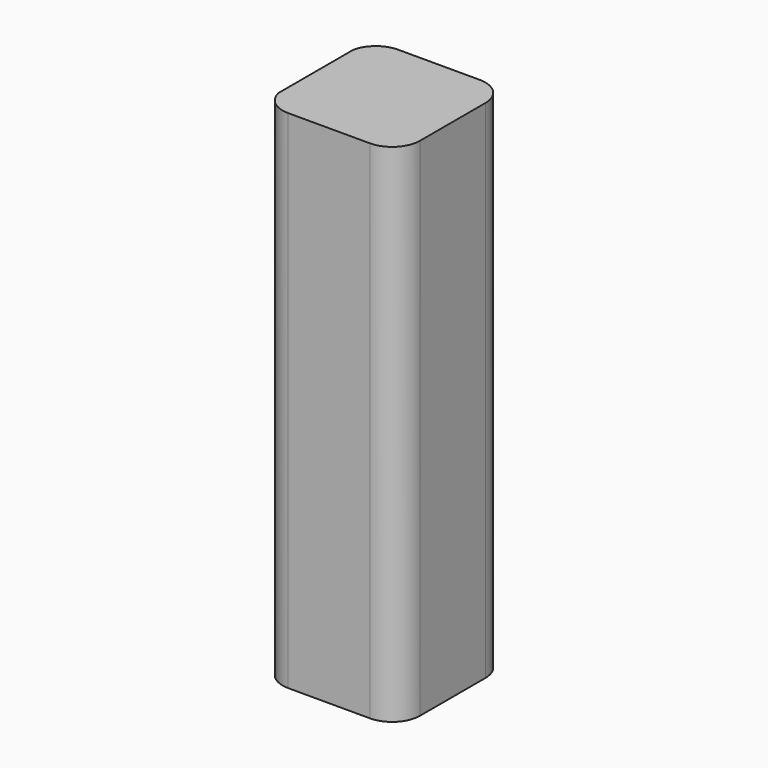
from build123d import *

# Parameters (mm, degrees)
F0_W         = 80
F0_H         = 60
F1_DEPTH     = 130
F2_T         = -1.5
F3_W         = 1.5
F3_H         = 27
F4_DEPTH     = 91
F5_R         = 1
F6_W         = 17
F6_H         = 16
F6_W_2       = 1.5
F6_H_2       = 27
F7_DEPTH     = 2
F8_T1_DEPTH  = 92
F8_T3_DEPTH  = 29.9726896882
F8_S7_W      = 1
F8_S7_H      = 1
F8_T8_DEPTH  = 1
F8_T15_DEPTH = 29.9726896882
F8_T19_DEPTH = 94.5
F9_T1_DEPTH  = 127.5
F9_T3_DEPTH  = 58.5
F9_S7_W      = 1
F9_S7_H      = 1
F9_T8_DEPTH  = 1
F9_S13_W     = 1
F9_S13_H     = 1
F9_T14_DEPTH = 1
F9_T18_ANGLE = 90
F11_DEPTH    = 60
F12_DEPTH    = 60
F13_DEPTH    = 50
F14_R        = 2
F15_W        = 17
F15_H        = 16
F16_DEPTH    = 91


# Not quite as in the source:
# - a fillet or chamfer that OpenCascade refuses, or shapes differently, is made with other operations: its cross-section is extruded or revolved along the edge and cut away or added


with BuildPart() as f1:
    # F0 (on Top) → F1 (new body)
    with BuildSketch(Plane.XY):
        Rectangle(F0_W, F0_H)
    extrude(amount=F1_DEPTH)

    # F2
    f2_openings = [f1.faces().sort_by_distance(p)[0] for p in [
        (0, 0, 130),
    ]]
    offset(amount=F2_T, openings=f2_openings)

    # F3 (on face) → F4 (join)
    with BuildSketch(Plane.XY.offset(1.5)):
        with Locations((11.75, -15)):
            Rectangle(F3_W, F3_H)
    extrude(amount=F4_DEPTH)

    # F5
    f5_edges = [f1.edges().sort_by_distance(p)[0] for p in [
        (0, 28.5, 1.5),
        (-38.5, 0, 1.5),
        (-13.75, -28.5, 1.5),
        (11, -15, 1.5),
    ]]
    fillet(f5_edges, radius=F5_R)

    # F6 (on face) → F7 (join)
    with BuildSketch(Plane.XY.offset(92.5)):
        Polygon((38.4726896882, -1.5), (12.5, -1.5), (12.5, -28.5), (11, -28.5), (11, -28.532365337), (38.4726896882, -28.532365337), align=None)
        with Locations((24.7363448441, -15)):
            Rectangle(F6_W, F6_H, mode=Mode.SUBTRACT)
        with Locations((11.75, -15)):
            Rectangle(F6_W_2, F6_H_2)
    extrude(amount=F7_DEPTH)

    # F8: fillet of radius 1 on 2 edges, made by hand

    # F8_s2 → F8_t1 (join)
    with BuildSketch(Plane.XY.offset(2.5)):
        with BuildLine():
            ThreePointArc((10, -28.5), (10.7071067812, -28.2071067812), (11, -27.5))
            Line((11, -27.5), (11, -28.5))
            Line((11, -28.5), (10, -28.5))
        make_face()
    extrude(amount=F8_T1_DEPTH)

    # F8_s4 → F8_t3 (join)
    with BuildSketch(Plane.YZ.offset(11)):
        with BuildLine():
            ThreePointArc((-28.5, 95.5), (-28.2071067812, 94.7928932188), (-27.5, 94.5))
            Line((-27.5, 94.5), (-28.5, 94.5))
            Line((-28.5, 94.5), (-28.5, 95.5))
        make_face()
    extrude(amount=F8_T3_DEPTH)


with BuildPart() as f8_tool6:
    # F8_s7 → F8_t8 (new body)
    with BuildSketch(Plane.XZ.offset(27.5)):
        with Locations((10.5, 2)):
            Rectangle(F8_S7_W, F8_S7_H)
    extrude(amount=F8_T8_DEPTH)

    # F8_s9 → F8_t10 (revolve, cut)
    with BuildSketch(Plane(origin=(10, -27.5, 2.5), x_dir=(-0.7071067812, 0, 0.7071067812), z_dir=(0.7071067812, 0, 0.7071067812))):
        with BuildLine():
            ThreePointArc((0, -1), (1, 0), (0, 1))
            Line((0, 1), (0, -1))
        make_face()
    revolve(axis=Axis((10, -27.5, 2.5), (0, -1, 0)), mode=Mode.SUBTRACT)


with BuildPart() as f1_1:
    add(f1.part)

    # F8_t5: union F8_tool6
    add(f8_tool6.part)


with BuildPart() as f8_tool13:
    # F8_s14 → F8_t15 (new body)
    with BuildSketch(Plane.YZ.offset(8.5)):
        with BuildLine():
            ThreePointArc((-28.5, 95.5), (-28.2071067812, 94.7928932188), (-27.5, 94.5))
            Line((-27.5, 94.5), (-28.5, 94.5))
            Line((-28.5, 94.5), (-28.5, 95.5))
        make_face()
    extrude(amount=F8_T15_DEPTH)

    split(bisect_by=Plane.YZ.offset(11), keep=Keep.BOTTOM)


with BuildPart() as f8_tool17:
    # F8_s18 → F8_t19 (new body)
    with BuildSketch(Plane.XY.offset(97)):
        with BuildLine():
            ThreePointArc((10, -28.5), (10.7071067812, -28.2071067812), (11, -27.5))
            Line((11, -27.5), (11, -28.5))
            Line((11, -28.5), (10, -28.5))
        make_face()
    extrude(amount=-F8_T19_DEPTH)

    split(bisect_by=Plane.XY.offset(94.5), keep=Keep.TOP)


with BuildPart() as f8_tool13_1:
    add(f8_tool13.part)

    # F8_t21: intersect F8_tool17
    add(f8_tool17.part, mode=Mode.INTERSECT)


with BuildPart() as f1_2:
    add(f1_1.part)

    # F8_t11: union F8_tool13
    add(f8_tool13_1.part)

    # F9: fillet of radius 1 on 3 edges, made by hand

    # F9_s2 → F9_t1 (join)
    with BuildSketch(Plane.XY.offset(2.5)):
        with BuildLine():
            ThreePointArc((-37.5, -28.5), (-38.2071067812, -28.2071067812), (-38.5, -27.5))
            Line((-38.5, -27.5), (-38.5, -28.5))
            Line((-38.5, -28.5), (-37.5, -28.5))
        make_face()
        with BuildLine():
            ThreePointArc((-37.5, 28.5), (-38.2071067812, 28.2071067812), (-38.5, 27.5))
            Line((-38.5, 27.5), (-38.5, 28.5))
            Line((-38.5, 28.5), (-37.5, 28.5))
        make_face()
        with BuildLine():
            ThreePointArc((37.5, 28.5), (38.2071067812, 28.2071067812), (38.5, 27.5))
            Line((38.5, 27.5), (38.5, 28.5))
            Line((38.5, 28.5), (37.5, 28.5))
        make_face()
    extrude(amount=F9_T1_DEPTH)

    # F9_s4 → F9_t3 (join)
    with BuildSketch(Plane.XZ.offset(-27.5)):
        with BuildLine():
            ThreePointArc((38.5, 2.5), (38.2071067812, 1.7928932188), (37.5, 1.5))
            Line((37.5, 1.5), (38.5, 1.5))
            Line((38.5, 1.5), (38.5, 2.5))
        make_face()
    extrude(amount=F9_T3_DEPTH)


with BuildPart() as f9_tool6:
    # F9_s7 → F9_t8 (new body)
    with BuildSketch(Plane.XZ.offset(-27.5)):
        with Locations((-38, 2)):
            Rectangle(F9_S7_W, F9_S7_H)
    extrude(amount=-F9_T8_DEPTH)

    # F9_s9 → F9_t10 (revolve, cut)
    with BuildSketch(Plane(origin=(-37.5, 27.5, 2.5), x_dir=(0.7071067812, 0, 0.7071067812), z_dir=(-0.7071067812, 0, 0.7071067812))):
        with BuildLine():
            ThreePointArc((0, -1), (1, 0), (0, 1))
            Line((0, 1), (0, -1))
        make_face()
    revolve(axis=Axis((-37.5, 27.5, 2.5), (0, 1, 0)), mode=Mode.SUBTRACT)


with BuildPart() as f1_3:
    add(f1_2.part)

    # F9_t5: union F9_tool6
    add(f9_tool6.part)


with BuildPart() as f9_tool12:
    # F9_s13 → F9_t14 (new body)
    with BuildSketch(Plane.XZ.offset(27.5)):
        with Locations((-38, 2)):
            Rectangle(F9_S13_W, F9_S13_H)
    extrude(amount=F9_T14_DEPTH)

    # F9_s15 → F9_t16 (revolve, cut)
    with BuildSketch(Plane(origin=(-37.5, -27.5, 2.5), x_dir=(0.7071067812, 0, 0.7071067812), z_dir=(0.7071067812, 0, -0.7071067812))):
        with BuildLine():
            ThreePointArc((0, -1), (1, 0), (0, 1))
            Line((0, 1), (0, -1))
        make_face()
    revolve(axis=Axis((-37.5, -27.5, 2.5), (0, -1, 0)), mode=Mode.SUBTRACT)


with BuildPart() as f1_4:
    add(f1_3.part)

    # F9_t11: union F9_tool12
    add(f9_tool12.part)

    # F9_s17 → F9_t18 (revolve)
    with BuildSketch(Plane.XY.offset(2.5)):
        with BuildLine():
            ThreePointArc((38.5, 27.5), (38.2071067812, 28.2071067812), (37.5, 28.5))
            Line((37.5, 28.5), (38.5, 28.5))
            Line((38.5, 28.5), (38.5, 27.5))
        make_face()
    revolve(axis=Axis((38.5, 27.5, 2.5), (-1, 0, 0)), revolution_arc=F9_T18_ANGLE)

    # F10 (on face) → F11 (join)
    with BuildSketch(Plane(origin=(0, 30, 0), x_dir=(-1, 0, 0), z_dir=(0, 1, 0))):
        Polygon((-42.6013286531, 4), (-41.4004783891, 2.4006374993), (-42.6, 1.5), (-44.4770764343, 4), (-45, 4), (-45, 0), (-40, 0), (-40, 4), align=None)
    extrude(amount=-F11_DEPTH)

    # F10 (on face) → F12 (join)
    with BuildSketch(Plane(origin=(0, 30, 0), x_dir=(-1, 0, 0), z_dir=(0, 1, 0))):
        Polygon((-65.4174783693, 34.3878804557), (-64.0949453732, 32.6264537871), (-40, 32.6264537871), (-40, 35.6264537871), (-68, 35.6264537871), (-68, 32.6264537871), (-65.9706931543, 32.6264537871), (-66.6169999802, 33.4872429564), align=None)
    extrude(amount=-F12_DEPTH)

    # F14
    f14_edges = [f1_4.edges().sort_by_distance(p)[0] for p in [
        (40, 0, 35.626454),
        (40, 0, 4),
        (40, 0, 32.626454),
    ]]
    fillet(f14_edges, radius=F14_R)


with BuildPart() as f13:
    # F10 (on face) → F13 (new body)
    with BuildSketch(Plane(origin=(0, 30, 0), x_dir=(-1, 0, 0), z_dir=(0, 1, 0))):
        Polygon((-42.6, 1.5), (-41.4004783891, 2.4006374993), (-42.6013286531, 4), (-44.4770764343, 4), align=None)
        Polygon((-44.4770764343, 4), (-42.6013286531, 4), (-64.0949453732, 32.6264537871), (-65.9706931543, 32.6264537871), align=None)
        Polygon((-65.9706931543, 32.6264537871), (-64.0949453732, 32.6264537871), (-65.4174783693, 34.3878804557), (-66.6169999802, 33.4872429564), align=None)
    extrude(amount=-F13_DEPTH)


with BuildPart() as f16:
    # F15 (on face) → F16 (new body)
    with BuildSketch(Plane(origin=(0, 0, 92.5), x_dir=(1, 0, 0), z_dir=(0, 0, -1))):
        with BuildLine():
            ThreePointArc((12.5, 6.589983932), (14.2478802784, 3.7576947486), (17.3863448441, 2.65))
            Line((17.3863448441, 2.65), (32.0863448441, 2.65))
            ThreePointArc((32.0863448441, 2.65), (35.62187875, 4.1144660941), (37.0863448441, 7.65))
            Line((37.0863448441, 7.65), (37.0863448441, 22.35))
            ThreePointArc((37.0863448441, 22.35), (35.62187875, 25.8855339059), (32.0863448441, 27.35))
            Line((32.0863448441, 27.35), (17.3863448441, 27.35))
            ThreePointArc((17.3863448441, 27.35), (14.2478802784, 26.2423052514), (12.5, 23.410016068))
            Line((12.5, 23.410016068), (12.5, 6.589983932))
        make_face()
        with Locations((24.7363448441, 15)):
            Rectangle(F15_W, F15_H, mode=Mode.SUBTRACT)
        with Locations((24.7363448441, 15)):
            Rectangle(F15_W, F15_H)
    extrude(amount=F16_DEPTH)


solid = f16.part
